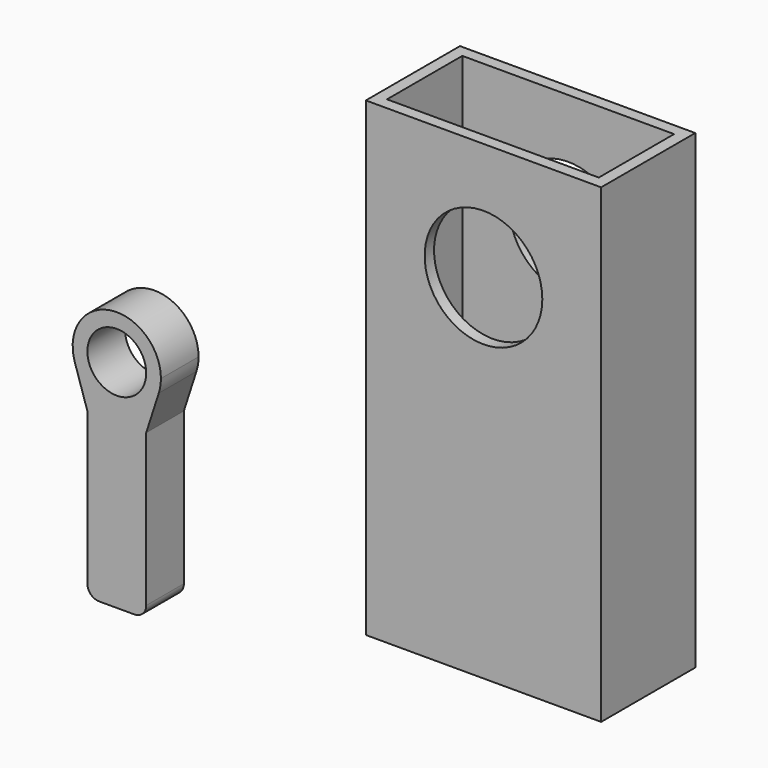
from build123d import *

# Parameters (mm, degrees)
F1_W     = 50.8
F1_H     = 25.4
F1_W_2   = 45.72
F1_H_2   = 20.3200011688
F2_DEPTH = 101.6
F3_R     = 12.7
F4_DEPTH = 25.4
F5_R     = 6.35
F6_DEPTH = 10.16


# Not quite as in the source:
# - a variable given as a bare number and used for a length is read in inches; the dataset says mm whatever the document's units were


with BuildPart() as f2:
    # F1 (on Top) → F2 (new body)
    with BuildSketch(Plane.XY):
        with Locations((12.6543196693, 2.8071403882)):
            Rectangle(F1_W, F1_H)
        with Locations((12.6543196693, 2.8071398037)):
            Rectangle(F1_W_2, F1_H_2, mode=Mode.SUBTRACT)
    extrude(amount=F2_DEPTH)

    # F3 (on face) → F4 (cut, through all)
    with BuildSketch(Plane.XZ.offset(9.8928596118)):
        with Locations((12.6543196693, 76.2)):
            Circle(F3_R)
    extrude(amount=-F4_DEPTH, mode=Mode.SUBTRACT)


with BuildPart() as f6:
    # F5 (on Front) → F6 (new body)
    with BuildSketch(Plane.XZ):
        with BuildLine():
            ThreePointArc((-56.7706652855, 34.5319435), (-67.7769258766, 43.9410609965), (-75.3599549571, 31.6054647715))
            ThreePointArc((-75.3599549571, 31.6054647715), (-66.2956652855, 25.0069435), (-57.2313756138, 31.6054647715))
            ThreePointArc((-57.2313756138, 31.6054647715), (-56.8865477891, 33.0506829089), (-56.7706652855, 34.5319435))
        make_face()
        with Locations((-66.2956652855, 34.5319435)):
            Circle(F5_R, mode=Mode.SUBTRACT)
        with BuildLine():
            Line((-75.3599549571, 31.6054647715), (-72.6456652855, 23.1983960315))
            Line((-72.6456652855, 23.1983960315), (-72.6456652855, -9.6236144723))
            ThreePointArc((-72.6456652855, -9.6236144723), (-71.9017165097, -11.4196656965), (-70.1056652855, -12.1636144723))
            Line((-70.1056652855, -12.1636144723), (-62.4856652855, -12.1636144723))
            ThreePointArc((-62.4856652855, -12.1636144723), (-60.6896140613, -11.4196656965), (-59.9456652855, -9.6236144723))
            Line((-59.9456652855, -9.6236144723), (-59.9456652855, 23.1983960315))
            Line((-59.9456652855, 23.1983960315), (-57.2313756138, 31.6054647715))
            ThreePointArc((-57.2313756138, 31.6054647715), (-66.2956652855, 25.0069435), (-75.3599549571, 31.6054647715))
        make_face()
    extrude(amount=F6_DEPTH)


solid = Compound([f2.part, f6.part])
